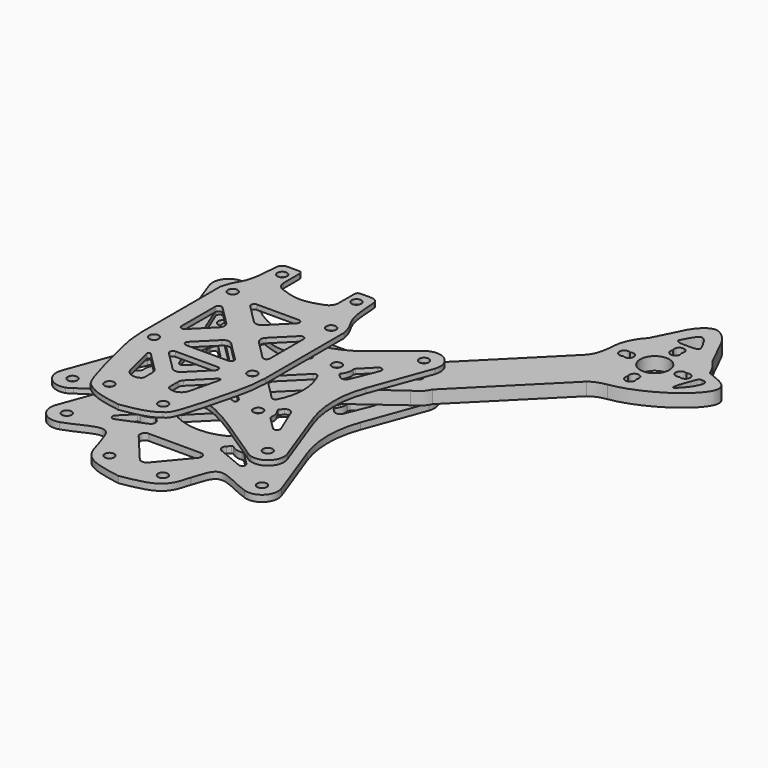
from build123d import *

# Parameters (mm, degrees)
F0_R     = 1.5
F2_DEPTH = 2
F4_START = 3
F1_R     = 1.5
F1_R_2   = 4.5
F4_DEPTH = 4
F7_START = 20
F6_R     = 1.5
F7_DEPTH = 1.5
F8_START = 9
F5_R     = 1.5
F8_DEPTH = 1.5


with BuildPart() as f2:
    # F0 (on Top) → F2 (new body)
    with BuildSketch(Plane.XY):
        with BuildLine():
            add(Edge.make_bspline(
                [(-28.6583371689, 34.989895508), (-15.5486081514, 28.1029236725), (-15.2531134537, 20.3288752095), (-15.0275822655, 35.7869570093)],
                knots=[0, 0, 0, 0, 13.3992828802, 13.3992828802, 13.3992828802, 13.3992828802], degree=3))
            ThreePointArc((-28.6583371689, 34.989895508), (-33.8221162144, 33.7485690999), (-34.9557615497, 28.560086322))
            Line((-34.9557615497, 28.560086322), (-28.2756954338, 10.3133747837))
            ThreePointArc((-28.2756954338, 10.3133747837), (-26.4471685044, -7.1088e-06), (-28.2756201348, -10.3134023513))
            Line((-28.2756201348, -10.3134023513), (-34.9643155344, -28.58409813))
            ThreePointArc((-34.9643155344, -28.58409813), (-33.8042341838, -33.7667341911), (-28.6341939914, -34.9817196608))
            add(Edge.make_bspline(
                [(-28.6341939914, -34.9817196608), (-24.495487875, -33.6930387827), (-16.3607874703, -27.7449542077), (-15.1366587225, -35.7631260416), (-14.33, -37.7577804035)],
                knots=[0, 0, 0, 0, 0.5615113554, 1, 1, 1, 1], degree=3))
            add(Edge.make_bspline(
                [(-14.33, -37.7577804035), (-13.6367446794, -40.3263257967), (-12.088150953, -46.0639424644), (-4.3010614265, -47.3817279873), (0, -48.1095835567)],
                knots=[0, 0, 0, 0, 0.447667654, 1, 1, 1, 1], degree=3))
            add(Edge.make_bspline(
                [(14.33, -37.7577804035), (13.6367446794, -40.3263257967), (12.088150953, -46.0639424644), (4.3010614265, -47.3817279873), (0, -48.1095835567)],
                knots=[0, 0, 0, 0, 0.447667654, 1, 1, 1, 1], degree=3))
            add(Edge.make_bspline(
                [(28.6583371689, -34.9898955092), (24.5097770544, -33.6967999), (16.3601661117, -27.7422129401), (15.1363049951, -35.7630085829), (14.33, -37.7577804035)],
                knots=[0, 0, 0, 0, 0.561784833, 1, 1, 1, 1], degree=3))
            ThreePointArc((28.6583371689, -34.9898955092), (33.8221162144, -33.748569101), (34.9557615497, -28.5600863232))
            Line((34.9557615497, -28.5600863232), (28.2756954338, -10.3133747849))
            ThreePointArc((28.2756954338, -10.3133747849), (26.4471685044, 7.1077e-06), (28.2756201348, 10.3134023502))
            Line((28.2756201348, 10.3134023502), (34.9643155344, 28.5840981288))
            ThreePointArc((34.9643155344, 28.5840981288), (33.8042341838, 33.76673419), (28.6341939914, 34.9817196596))
            add(Edge.make_bspline(
                [(15.0274820378, 35.7867377887), (15.2513136358, 20.3289797995), (15.5248044507, 28.1031931102), (28.6341939914, 34.9817196596)],
                knots=[0.5359060708, 0.5359060708, 0.5359060708, 0.5359060708, 13.9139411757, 13.9139411757, 13.9139411757, 13.9139411757], degree=3))
            ThreePointArc((15.0274820378, 35.7867377887), (14.4316299327, 37.1821951546), (13.0276916813, 37.7577804023))
            Line((13.0276916813, 37.7577804023), (-13.0277950954, 37.7577804023))
            ThreePointArc((-13.0277950954, 37.7577804023), (-14.4316552711, 37.1822721036), (-15.0275822655, 35.7869570093))
        make_face()
        with Locations((-30.25, -30.2500000006)):
            Circle(F0_R, mode=Mode.SUBTRACT)
        with Locations((-8.2733329443, -41.1618490551)):
            Circle(F0_R, mode=Mode.SUBTRACT)
        with BuildLine():
            ThreePointArc((-23.8517090122, -20.3161751069), (-25.1141961389, -20.4406647854), (-25.4828700073, -19.2268068843))
            Line((-25.4828700073, -19.2268068843), (-22.1833207357, -11.2506887671))
            ThreePointArc((-22.1833207357, -11.2506887671), (-21.0902108457, -10.3529698728), (-19.736579243, -10.7634207575))
            Line((-19.736579243, -10.7634207575), (-18.8553009264, -11.6446990741))
            ThreePointArc((-18.8553009264, -11.6446990741), (-18.7090370991, -11.9847340093), (-18.8367068235, -12.33217797))
            Line((-18.8367068235, -12.33217797), (-18.8542943682, -12.3517786311))
            ThreePointArc((-18.8542943682, -12.3517786311), (-19.6877326512, -13.9472514003), (-19.8489637612, -15.7400584892))
            Line((-19.8489637612, -15.7400584892), (-19.8303976916, -15.8549305034))
            ThreePointArc((-19.8303976916, -15.8549305034), (-19.8571321349, -16.2052315209), (-20.0404595752, -16.5049256699))
            Line((-20.0404595752, -16.5049256699), (-23.8517090122, -20.3161751069))
        make_face(mode=Mode.SUBTRACT)
        with BuildLine():
            Line((-11.2506887665, -22.1833207364), (-19.2268068836, -25.482870008))
            ThreePointArc((-19.2268068836, -25.482870008), (-20.4406647847, -25.1141961396), (-20.3161751062, -23.8517090128))
            Line((-20.3161751062, -23.8517090128), (-16.5049256693, -20.0404595759))
            ThreePointArc((-16.5049256693, -20.0404595759), (-16.2052315202, -19.8571321356), (-15.8549305027, -19.8303976923))
            Line((-15.8549305027, -19.8303976923), (-15.7400584885, -19.8489637619))
            ThreePointArc((-15.7400584885, -19.8489637619), (-13.9472513996, -19.6877326519), (-12.3517786304, -18.8542943689))
            Line((-12.3517786304, -18.8542943689), (-12.3321779693, -18.8367068242))
            ThreePointArc((-12.3321779693, -18.8367068242), (-11.9847340086, -18.7090370997), (-11.6446990734, -18.8553009271))
            Line((-11.6446990734, -18.8553009271), (-10.7634207569, -19.7365792436))
            ThreePointArc((-10.7634207569, -19.7365792436), (-10.3529698721, -21.0902108464), (-11.2506887665, -22.1833207364))
        make_face(mode=Mode.SUBTRACT)
        with Locations((-15.25, -15.2500000006)):
            Circle(F0_R, mode=Mode.SUBTRACT)
        with BuildLine():
            ThreePointArc((-7.7892382513, -15.2383616248), (-8.2896410828, -14.5053634666), (-8.0071487762, -13.6640030263))
            Line((-8.0071487762, -13.6640030263), (-1.4142135624, -7.0710678125))
            ThreePointArc((-1.4142135624, -7.0710678125), (0, -6.4852813748), (1.4142135624, -7.0710678125))
            Line((1.4142135624, -7.0710678125), (8.0039929944, -13.6608472445))
            ThreePointArc((8.0039929944, -13.6608472445), (8.287442711, -14.5050591849), (7.7853439372, -15.2405415869))
            Line((7.7853439372, -15.2405415869), (7.7684472975, -15.2500000006))
            ThreePointArc((7.7684472975, -15.2500000006), (0, -17.1146508417), (-7.7684472975, -15.2500000006))
            Line((-7.7684472975, -15.2500000006), (-7.7892382513, -15.2383616248))
        make_face(mode=Mode.SUBTRACT)
        with Locations((8.2733329443, -41.1618490551)):
            Circle(F0_R, mode=Mode.SUBTRACT)
        with BuildLine():
            Line((-1.3419338656, -38.0910861377), (-9.1892168108, -28.7161126104))
            ThreePointArc((-9.1892168108, -28.7161126104), (-9.3980668278, -27.118570832), (-8.0389877832, -26.2533181443))
            Line((-8.0389877832, -26.2533181443), (8.0389877833, -26.2533181443))
            ThreePointArc((8.0389877833, -26.2533181443), (9.398066828, -27.118570832), (9.189216811, -28.7161126104))
            Line((9.189216811, -28.7161126104), (1.3419338656, -38.0910861377))
            ThreePointArc((1.3419338656, -38.0910861377), (0, -38.7178259272), (-1.3419338656, -38.0910861377))
        make_face(mode=Mode.SUBTRACT)
        with Locations((30.25, -30.2500000006)):
            Circle(F0_R, mode=Mode.SUBTRACT)
        with BuildLine():
            ThreePointArc((20.3161751064, -23.8517090128), (20.4406647849, -25.1141961396), (19.2268068838, -25.482870008))
            Line((19.2268068838, -25.482870008), (11.2506887667, -22.1833207364))
            ThreePointArc((11.2506887667, -22.1833207364), (10.3529698723, -21.0902108464), (10.7634207571, -19.7365792436))
            Line((10.7634207571, -19.7365792436), (11.6446990736, -18.8553009271))
            ThreePointArc((11.6446990736, -18.8553009271), (11.9847340088, -18.7090370997), (12.3321779695, -18.8367068242))
            Line((12.3321779695, -18.8367068242), (12.3517786306, -18.8542943689))
            ThreePointArc((12.3517786306, -18.8542943689), (13.9472513998, -19.6877326519), (15.7400584887, -19.8489637619))
            Line((15.7400584887, -19.8489637619), (15.8549305029, -19.8303976923))
            ThreePointArc((15.8549305029, -19.8303976923), (16.2052315204, -19.8571321356), (16.5049256694, -20.0404595759))
            Line((16.5049256694, -20.0404595759), (20.3161751064, -23.8517090128))
        make_face(mode=Mode.SUBTRACT)
        with Locations((15.25, -15.2500000006)):
            Circle(F0_R, mode=Mode.SUBTRACT)
        with BuildLine():
            ThreePointArc((19.7365792431, -10.7634207575), (21.0902108459, -10.3529698728), (22.1833207359, -11.2506887671))
            Line((22.1833207359, -11.2506887671), (25.4828700075, -19.2268068842))
            ThreePointArc((25.4828700075, -19.2268068842), (25.1141961391, -20.4406647853), (23.8517090123, -20.3161751069))
            Line((23.8517090123, -20.3161751069), (20.0404595754, -16.5049256699))
            ThreePointArc((20.0404595754, -16.5049256699), (19.8571321351, -16.2052315209), (19.8303976918, -15.8549305033))
            Line((19.8303976918, -15.8549305033), (19.8489637614, -15.7400584892))
            ThreePointArc((19.8489637614, -15.7400584892), (19.6877326514, -13.9472514003), (18.8542943684, -12.3517786311))
            Line((18.8542943684, -12.3517786311), (18.8367068237, -12.33217797))
            ThreePointArc((18.8367068237, -12.33217797), (18.7090370992, -11.9847340093), (18.8553009266, -11.6446990741))
            Line((18.8553009266, -11.6446990741), (19.7365792431, -10.7634207575))
        make_face(mode=Mode.SUBTRACT)
        with BuildLine():
            ThreePointArc((-18.8367068237, 12.3321779688), (-18.7090370992, 11.9847340081), (-18.8553009266, 11.6446990729))
            Line((-18.8553009266, 11.6446990729), (-19.7365318181, 10.7634681813))
            ThreePointArc((-19.7365318181, 10.7634681813), (-21.0901735727, 10.3530193183), (-22.1832812244, 11.250755321))
            Line((-22.1832812244, 11.250755321), (-25.4825410679, 19.2264854211))
            ThreePointArc((-25.4825410679, 19.2264854211), (-25.1138561851, 20.4403344014), (-23.851374797, 20.3158408904))
            Line((-23.851374797, 20.3158408904), (-20.0404595754, 16.5049256687))
            ThreePointArc((-20.0404595754, 16.5049256687), (-19.8571321351, 16.2052315197), (-19.8303976918, 15.8549305022))
            Line((-19.8303976918, 15.8549305022), (-19.8489637614, 15.740058488))
            ThreePointArc((-19.8489637614, 15.740058488), (-19.6877326514, 13.9472513991), (-18.8542943684, 12.3517786299))
            Line((-18.8542943684, 12.3517786299), (-18.8367068237, 12.3321779688))
        make_face(mode=Mode.SUBTRACT)
        with BuildLine():
            ThreePointArc((-13.6608472446, -8.003992994), (-14.505059185, -8.2874427105), (-15.2405415869, -7.7853439367))
            Line((-15.2405415869, -7.7853439367), (-15.25, -7.7684472983))
            ThreePointArc((-15.25, -7.7684472983), (-17.1146508411, -6e-10), (-15.25, 7.7684472971))
            Line((-15.25, 7.7684472971), (-15.2405415859, 7.7853439372))
            ThreePointArc((-15.2405415859, 7.7853439372), (-14.505059184, 8.2874427111), (-13.6608472436, 8.0039929945))
            Line((-13.6608472436, 8.0039929945), (-7.0710678122, 1.4142135631))
            ThreePointArc((-7.0710678122, 1.4142135631), (-6.4852813746, 7e-10), (-7.0710678122, -1.4142135616))
            Line((-7.0710678122, -1.4142135616), (-13.6608472446, -8.003992994))
        make_face(mode=Mode.SUBTRACT)
        with Locations((-15.25, 15.2499999994)):
            Circle(F0_R, mode=Mode.SUBTRACT)
        with BuildLine():
            ThreePointArc((7.7853439372, 15.2405415857), (8.287442711, 14.5050591838), (8.0039929944, 13.6608472433))
            Line((8.0039929944, 13.6608472433), (1.4142135624, 7.0710678113))
            ThreePointArc((1.4142135624, 7.0710678113), (0, 6.4852813737), (-1.4142135624, 7.0710678113))
            Line((-1.4142135624, 7.0710678113), (-8.0039929944, 13.6608472433))
            ThreePointArc((-8.0039929944, 13.6608472433), (-8.287442711, 14.5050591838), (-7.7853439372, 15.2405415857))
            Line((-7.7853439372, 15.2405415857), (-7.7684472975, 15.2499999994))
            ThreePointArc((-7.7684472975, 15.2499999994), (0, 17.1146508406), (7.7684472975, 15.2499999994))
            Line((7.7684472975, 15.2499999994), (7.7853439372, 15.2405415857))
        make_face(mode=Mode.SUBTRACT)
        with Locations((-30.25, 30.2499999994)):
            Circle(F0_R, mode=Mode.SUBTRACT)
        with BuildLine():
            ThreePointArc((-7.7684472975, 20.1190513336), (-9.4080907996, 20.7386520685), (-8.9382902045, 22.4273270773))
            Line((-8.9382902045, 22.4273270773), (-1.06072927, 27.355528746))
            ThreePointArc((-1.06072927, 27.355528746), (0, 27.6599894761), (1.0607292699, 27.355528746))
            Line((1.0607292699, 27.355528746), (8.9382902045, 22.4273270773))
            ThreePointArc((8.9382902045, 22.4273270773), (9.4121452662, 20.7467816187), (7.7853439372, 20.1125189809))
            ThreePointArc((7.7853439372, 20.1125189809), (0.0090577048, 21.5667549236), (-7.7684472975, 20.1190513336))
        make_face(mode=Mode.SUBTRACT)
        with Locations((-11.5, 29.7577804023)):
            Circle(F0_R, mode=Mode.SUBTRACT)
        with BuildLine():
            Line((7.0710678124, 1.4142135624), (13.6608472439, 8.0039929938))
            ThreePointArc((13.6608472439, 8.0039929938), (14.5050591843, 8.2874427104), (15.2405415863, 7.7853439366))
            Line((15.2405415863, 7.7853439366), (15.25, 7.7684472971))
            ThreePointArc((15.25, 7.7684472971), (17.1146508411, -6e-10), (15.25, -7.7684472983))
            Line((15.25, -7.7684472983), (15.2405415867, -7.7853439371))
            ThreePointArc((15.2405415867, -7.7853439371), (14.5050591848, -8.2874427109), (13.6608472444, -8.0039929943))
            Line((13.6608472444, -8.0039929943), (7.0710678124, -1.4142135624))
            ThreePointArc((7.0710678124, -1.4142135624), (6.4852813748, 0), (7.0710678124, 1.4142135624))
        make_face(mode=Mode.SUBTRACT)
        with Locations((15.25, 15.2499999994)):
            Circle(F0_R, mode=Mode.SUBTRACT)
        with BuildLine():
            Line((19.8247048971, 15.785759925), (19.8053184489, 15.9004963368))
            ThreePointArc((19.8053184489, 15.9004963368), (19.8295490283, 16.2509794496), (20.0107302331, 16.5519759685))
            Line((20.0107302331, 16.5519759685), (23.8084562188, 20.4043695836))
            ThreePointArc((23.8084562188, 20.4043695836), (25.0693920791, 20.5382911332), (25.4479247727, 19.3280815542))
            Line((25.4479247727, 19.3280815542), (22.2099579078, 11.3050038785))
            ThreePointArc((22.2099579078, 11.3050038785), (21.1235499455, 10.3976310998), (19.7659136105, 10.7981697397))
            Line((19.7659136105, 10.7981697397), (18.8636878016, 11.6875924575))
            ThreePointArc((18.8636878016, 11.6875924575), (18.7150078324, 12.0262851571), (18.8397994936, 12.37448843))
            Line((18.8397994936, 12.37448843), (18.8575858105, 12.3946446988))
            ThreePointArc((18.8575858105, 12.3946446988), (19.6770217108, 13.9944130467), (19.8247048971, 15.785759925))
        make_face(mode=Mode.SUBTRACT)
        with Locations((11.5, 29.7577804023)):
            Circle(F0_R, mode=Mode.SUBTRACT)
        with Locations((30.25, 30.2499999994)):
            Circle(F0_R, mode=Mode.SUBTRACT)
    extrude(amount=F2_DEPTH)


with BuildPart() as f4:
    # F1 (on Top) → F4 (new body)
    with BuildSketch(Plane.XY.offset(F4_START)):
        with BuildLine():
            add(Edge.make_bspline(
                [(53.8403756487, 63.7304752458), (55.416769934, 65.2037108877), (56.4797969246, 66.7322054505), (56.9693953395, 70.96)],
                knots=[0, 0, 0, 0, 7.8776133694, 7.8776133694, 7.8776133694, 7.8776133694], degree=3))
            Line((53.8403756487, 63.7304752458), (27.2135911477, 37.1036907448))
            ThreePointArc((27.2135911477, 37.1036907448), (24.9560944806, 35.5533008589), (23.4057045947, 33.2958041918))
            Line((23.4057045947, 33.2958041918), (13.6185183249, 19.9730840161))
            ThreePointArc((13.6185183249, 19.9730840161), (11.3998018999, 18.428606374), (10.3093393921, 15.9549440526))
            Line((10.3093393921, 15.9549440526), (6.3693953395, 12.015))
            Line((6.3693953395, 12.015), (0.0093953395, 5.655))
            Line((0.0093953395, 5.655), (0.0093953395, 0))
            Line((0.0093953395, 0), (5.6643953395, 0))
            Line((5.6643953395, 0), (12.0243953395, 6.36))
            Line((12.0243953395, 6.36), (15.964339392, 10.2999440526))
            ThreePointArc((15.964339392, 10.2999440526), (18.4380017135, 11.3904065604), (19.9824793556, 13.6091229854))
            Line((19.9824793556, 13.6091229854), (33.3051995313, 23.3963092552))
            ThreePointArc((33.3051995313, 23.3963092552), (35.5626961984, 24.9466991411), (37.1130860843, 27.2041958082))
            Line((37.1130860843, 27.2041958082), (63.6551645076, 53.7462742315))
            add(Edge.make_bspline(
                [(63.6551645076, 53.7462742315), (65.3627067804, 54.9906902015), (66.7258799076, 55.3231723607), (68.4891356677, 55.6597283697)],
                knots=[0, 0, 0, 0, 5.1989021836, 5.1989021836, 5.1989021836, 5.1989021836], degree=3))
            add(Edge.make_bspline(
                [(84.0894447875, 75.8451102834), (87.0090253606, 74.6406662064), (97.809192454, 71.4575524374), (79.1750401258, 57.3118105531), (68.4891356677, 55.6597283697)],
                knots=[0, 0, 0, 0, 0.3577567319, 1, 1, 1, 1], degree=3))
            ThreePointArc((84.0894447875, 75.8451102834), (82.7490756952, 78.5256546787), (80.8688902761, 80.8594949366))
            Line((80.8688902761, 80.8594949366), (76.2193953395, 90.2586398484))
            add(Edge.make_bspline(
                [(65.7193953395, 90.2586398484), (67.2193953395, 92.6020138718), (70.9693953395, 96.3179861282), (74.7193953395, 92.6020138718), (76.2193953395, 90.2586398484)],
                knots=[0, 0, 0, 0, 0.5, 1, 1, 1, 1], degree=3))
            Line((65.7193953395, 90.2586398484), (61.0699004029, 80.8594949366))
            ThreePointArc((61.0699004029, 80.8594949366), (58.0350818843, 76.3175680531), (56.9693953395, 70.96))
        make_face()
        with Locations((15.2593953395, 15.25)):
            Circle(F1_R, mode=Mode.SUBTRACT)
        with Locations((30.2593953395, 30.25)):
            Circle(F1_R, mode=Mode.SUBTRACT)
        with BuildLine():
            ThreePointArc((72.2684334452, 62.21), (70.9693953395, 59.96), (69.6703572338, 62.21))
            ThreePointArc((69.6703572338, 62.21), (70.9693953395, 64.46), (72.2684334452, 62.21))
        make_face(mode=Mode.SUBTRACT)
        with BuildLine():
            ThreePointArc((62.2193953395, 72.2590381057), (64.4693953395, 70.96), (62.2193953395, 69.6609618943))
            ThreePointArc((62.2193953395, 69.6609618943), (59.9693953395, 70.96), (62.2193953395, 72.2590381057))
        make_face(mode=Mode.SUBTRACT)
        with Locations((70.9693953395, 70.96)):
            Circle(F1_R_2, mode=Mode.SUBTRACT)
        with BuildLine():
            add(Edge.make_bspline(
                [(82.4060514569, 64.5534098148), (80.7914603636, 63.0556593791), (83.9801204568, 71.8950702465), (84.2074600213, 71.8239934193), (84.9451732404, 71.783184101)],
                knots=[0, 0, 0, 0, 0.6805312174, 1, 1, 1, 1], degree=3))
            add(Edge.make_bspline(
                [(84.9451732404, 71.783184101), (85.7962933376, 71.6849426877), (87.6041236849, 71.2964912458), (84.6678863419, 66.376809069), (82.4060514569, 64.5534098148)],
                knots=[0, 0, 0, 0, 0.32334118, 1, 1, 1, 1], degree=3))
        make_face(mode=Mode.SUBTRACT)
        with BuildLine():
            ThreePointArc((79.7193953395, 69.6609618943), (77.4693953395, 70.96), (79.7193953395, 72.2590381057))
            ThreePointArc((79.7193953395, 72.2590381057), (81.9693953395, 70.96), (79.7193953395, 69.6609618943))
        make_face(mode=Mode.SUBTRACT)
        with BuildLine():
            ThreePointArc((72.2684334452, 79.71), (70.9693953395, 77.46), (69.6703572338, 79.71))
            ThreePointArc((69.6703572338, 79.71), (70.9693953395, 81.96), (72.2684334452, 79.71))
        make_face(mode=Mode.SUBTRACT)
        with BuildLine():
            add(Edge.make_bspline(
                [(67.4763052703, 84.5172239698), (67.595660109, 83.524372308), (70.9693953395, 83.524372308), (74.34313057, 83.524372308), (74.4624854087, 84.5172239698)],
                knots=[0, 0, 0, 0, 0.5, 1, 1, 1, 1], degree=3))
            add(Edge.make_bspline(
                [(67.4763052703, 84.5172239698), (68.6406686267, 86.8665499989), (70.9693953395, 91.5652020569), (73.2981220523, 86.8665499989), (74.4624854087, 84.5172239698)],
                knots=[0, 0, 0, 0, 0.5, 1, 1, 1, 1], degree=3))
        make_face(mode=Mode.SUBTRACT)
    extrude(amount=F4_DEPTH)


with BuildPart() as f7:
    # F6 (on Top) → F7 (new body)
    with BuildSketch(Plane.XY.offset(F7_START)):
        with BuildLine():
            add(Edge.make_bspline(
                [(-19.25, -15.2218541075), (-19.0684905374, -19.7268529833), (-17.9623264747, -24.6907042809), (-13.2785718821, -43.084666195), (-11.6053951728, -44.1968771124), (-11.0003547743, -44.5749795424)],
                knots=[0, 0, 0, 0, 0.3683029461, 0.8298524693, 1, 1, 1, 1], degree=3))
            add(Edge.make_bspline(
                [(-11.0003547743, -44.5749795424), (-7.8986920416, -46.9837644324), (-3.9995196275, -47.3454079802), (0, -48.1093942399)],
                knots=[0, 0, 0, 0, 11.5542153526, 11.5542153526, 11.5542153526, 11.5542153526], degree=3))
            add(Edge.make_bspline(
                [(11.0003547743, -44.5749795424), (7.8986920416, -46.9837644324), (3.9995196275, -47.3454079802), (0, -48.1093942399)],
                knots=[0, 0, 0, 0, 11.5542153526, 11.5542153526, 11.5542153526, 11.5542153526], degree=3))
            add(Edge.make_bspline(
                [(19.25, -15.2218541075), (19.0667337669, -19.7267716154), (17.9562925595, -24.6902276301), (13.2790290127, -43.0847539077), (11.6055152346, -44.1969091306), (11.0003547743, -44.5749795424)],
                knots=[0, 0, 0, 0, 0.368314136, 0.829851714, 1, 1, 1, 1], degree=3))
            Line((19.25, -15.2218541075), (19.25, 15.2781458925))
            add(Edge.make_bspline(
                [(15.0790967662, 31.8597836794), (15.7273210805, 18.4148469189), (17.670676786, 22.4575338068), (19.25, 15.2781458925)],
                knots=[0.8128411452, 0.8128411452, 0.8128411452, 0.8128411452, 18.97635654, 18.97635654, 18.97635654, 18.97635654], degree=3))
            ThreePointArc((15.0790967662, 31.8597836794), (14.4611582834, 33.211334576), (13.0814172406, 33.7634690247))
            add(Edge.make_bspline(
                [(9.5020394819, 33.7713114856), (10.6902314797, 33.7688881845), (11.9558724743, 33.7634690247), (13.0814172406, 33.7634690247)],
                knots=[1.0243447025, 1.0243447025, 1.0243447025, 1.0243447025, 4.5814260604, 4.5814260604, 4.5814260604, 4.5814260604], degree=3))
            ThreePointArc((9.5020394819, 33.7713114856), (8.7936146526, 33.479141045), (8.5, 32.7713135654))
            add(Edge.make_bspline(
                [(8.5, 32.285449478), (8.5, 32.4472244474), (8.5, 32.609243629), (8.5, 32.7713135654)],
                knots=[0.2605482636, 0.2605482636, 0.2605482636, 0.2605482636, 0.7461719983, 0.7461719983, 0.7461719983, 0.7461719983], degree=3))
            add(Edge.make_bspline(
                [(8.5, 32.025302314), (8.5, 32.1119278185), (8.5, 32.1986534992), (8.5, 32.285449478)],
                knots=[0, 0, 0, 0, 0.2605482636, 0.2605482636, 0.2605482636, 0.2605482636], degree=3))
            Line((8.5, 32.025302314), (8.5, 26.5908181775))
            ThreePointArc((8.5, 26.5908181775), (7.9671627129, 24.8840351954), (6.5579279014, 23.7835439559))
            add(Edge.make_bspline(
                [(-6.5579279014, 23.7835439559), (-4.3358517051, 22.9461493085), (0, 21.578151535), (4.3358517051, 22.9461493085), (6.5579279014, 23.7835439559)],
                knots=[0.1121315865, 0.1121315865, 0.1121315865, 0.1121315865, 0.5, 0.8878684135, 0.8878684135, 0.8878684135, 0.8878684135], degree=3))
            ThreePointArc((-6.5579279014, 23.7835439559), (-7.9671627129, 24.8840351954), (-8.5, 26.5908181775))
            Line((-8.5, 26.5908181775), (-8.5, 32.025302314))
            add(Edge.make_bspline(
                [(-8.5, 32.025302314), (-8.5, 32.1119278185), (-8.5, 32.1986534992), (-8.5, 32.285449478)],
                knots=[0, 0, 0, 0, 0.2605482636, 0.2605482636, 0.2605482636, 0.2605482636], degree=3))
            add(Edge.make_bspline(
                [(-8.5, 32.285449478), (-8.5, 32.4469519552), (-8.5, 32.6086978226), (-8.5, 32.7704945986)],
                knots=[0.2605482636, 0.2605482636, 0.2605482636, 0.2605482636, 0.7453540183, 0.7453540183, 0.7453540183, 0.7453540183], degree=3))
            ThreePointArc((-8.5, 32.7704945986), (-8.7935873047, 33.4782947851), (-9.501962208, 33.7704926735))
            Line((-9.501962208, 33.7704926735), (-13.0814172406, 33.7634690247))
            ThreePointArc((-13.0814172406, 33.7634690247), (-14.4611582834, 33.211334576), (-15.0790967662, 31.8597836794))
            add(Edge.make_bspline(
                [(-15.0790967662, 31.8597836794), (-15.7273210805, 18.4148469189), (-17.670676786, 22.4575338068), (-19.25, 15.2781458925)],
                knots=[0.8128411452, 0.8128411452, 0.8128411452, 0.8128411452, 18.97635654, 18.97635654, 18.97635654, 18.97635654], degree=3))
            Line((-19.25, 15.2781458925), (-19.25, -15.2218541075))
        make_face()
        with Locations((-8.3293477558, -41.1257331912)):
            Circle(F6_R, mode=Mode.SUBTRACT)
        with BuildLine():
            ThreePointArc((-11.2741795299, -22.9536277928), (-11.0338873267, -22.3989447209), (-10.4349964383, -22.4810626653))
            Line((-10.4349964383, -22.4810626653), (-4.5076118446, -28.408447259))
            ThreePointArc((-4.5076118446, -28.408447259), (-4.0740663419, -29.0572939567), (-3.9218254069, -29.8226608214))
            Line((-3.9218254069, -29.8226608214), (-3.9218254069, -32.9968597055))
            ThreePointArc((-3.9218254069, -32.9968597055), (-4.0264596985, -33.4421913215), (-4.3184659033, -33.7943290211))
            Line((-4.3184659033, -33.7943290211), (-4.4003069963, -33.8562493989))
            ThreePointArc((-4.4003069963, -33.8562493989), (-7.223873087, -34.0855754205), (-9.0722171951, -31.9387778169))
            Line((-9.0722171951, -31.9387778169), (-11.2741795299, -22.9536277928))
        make_face(mode=Mode.SUBTRACT)
        with Locations((-15.25, -15.2218541075)):
            Circle(F6_R, mode=Mode.SUBTRACT)
        with Locations((8.3288047093, -41.1259644251)):
            Circle(F6_R, mode=Mode.SUBTRACT)
        with BuildLine():
            Line((4.5076118446, -28.408447259), (10.4349123369, -22.4811467667))
            ThreePointArc((10.4349123369, -22.4811467667), (11.0338107336, -22.3990330505), (11.2740913261, -22.9537286326))
            Line((11.2740913261, -22.9537286326), (9.0718254069, -31.9387778169))
            ThreePointArc((9.0718254069, -31.9387778169), (7.2237469097, -34.0856955052), (4.4002690575, -33.8562995378))
            Line((4.4002690575, -33.8562995378), (4.3183823385, -33.7943311455))
            ThreePointArc((4.3183823385, -33.7943311455), (4.0264363662, -33.4422097633), (3.9218254069, -32.9969250614))
            Line((3.9218254069, -32.9969250614), (3.9218254069, -29.8226608214))
            ThreePointArc((3.9218254069, -29.8226608214), (4.0740663419, -29.0572939567), (4.5076118446, -28.408447259))
        make_face(mode=Mode.SUBTRACT)
        with BuildLine():
            Line((-1.4142135624, -25.3091152098), (-7.2178932188, -19.5054355534))
            ThreePointArc((-7.2178932188, -19.5054355534), (-7.4346659701, -18.4156453398), (-6.5107864376, -17.7983287722))
            Line((-6.5107864376, -17.7983287722), (6.5107864376, -17.7983287722))
            ThreePointArc((6.5107864376, -17.7983287722), (7.4346659701, -18.4156453398), (7.2178932188, -19.5054355534))
            Line((7.2178932188, -19.5054355534), (1.4142135624, -25.3091152098))
            ThreePointArc((1.4142135624, -25.3091152098), (0, -25.8949016474), (-1.4142135624, -25.3091152098))
        make_face(mode=Mode.SUBTRACT)
        with BuildLine():
            ThreePointArc((-1.4142135624, -6.1360676699), (0, -5.5502812323), (1.4142135624, -6.1360676699))
            Line((1.4142135624, -6.1360676699), (7.2178932188, -11.9397473263))
            ThreePointArc((7.2178932188, -11.9397473263), (7.4346659701, -13.0295375399), (6.5107864376, -13.6468541075))
            Line((6.5107864376, -13.6468541075), (-6.5107864376, -13.6468541075))
            ThreePointArc((-6.5107864376, -13.6468541075), (-7.4346659701, -13.0295375399), (-7.2178932188, -11.9397473263))
            Line((-7.2178932188, -11.9397473263), (-1.4142135624, -6.1360676699))
        make_face(mode=Mode.SUBTRACT)
        with Locations((15.25, -15.2218541075)):
            Circle(F6_R, mode=Mode.SUBTRACT)
        with BuildLine():
            Line((-11.9678932188, 7.2460391113), (-6.1642135624, 1.4423594549))
            ThreePointArc((-6.1642135624, 1.4423594549), (-5.5784271247, 0.0281458925), (-6.1642135624, -1.3860676699))
            Line((-6.1642135624, -1.3860676699), (-11.9678932188, -7.1897473263))
            ThreePointArc((-11.9678932188, -7.1897473263), (-13.0576834324, -7.4065200777), (-13.675, -6.4826405451))
            Line((-13.675, -6.4826405451), (-13.675, 6.5389323301))
            ThreePointArc((-13.675, 6.5389323301), (-13.0576834324, 7.4628118626), (-11.9678932188, 7.2460391113))
        make_face(mode=Mode.SUBTRACT)
        with Locations((-15.25, 15.2781458925)):
            Circle(F6_R, mode=Mode.SUBTRACT)
        with Locations((-11.499689569, 29.7634854823)):
            Circle(F6_R, mode=Mode.SUBTRACT)
        with BuildLine():
            ThreePointArc((1.4142135624, 6.1923594549), (0, 5.6065730172), (-1.4142135624, 6.1923594549))
            Line((-1.4142135624, 6.1923594549), (-7.2178932188, 11.9960391113))
            ThreePointArc((-7.2178932188, 11.9960391113), (-7.4346659701, 13.0858293249), (-6.5107864376, 13.7031458925))
            Line((-6.5107864376, 13.7031458925), (6.5107864376, 13.7031458925))
            ThreePointArc((6.5107864376, 13.7031458925), (7.4346659701, 13.0858293249), (7.2178932188, 11.9960391113))
            Line((7.2178932188, 11.9960391113), (1.4142135624, 6.1923594549))
        make_face(mode=Mode.SUBTRACT)
        with BuildLine():
            Line((11.9678932188, -7.1897473263), (6.1642135624, -1.3860676699))
            ThreePointArc((6.1642135624, -1.3860676699), (5.5784271247, 0.0281458925), (6.1642135624, 1.4423594549))
            Line((6.1642135624, 1.4423594549), (11.9678932188, 7.2460391113))
            ThreePointArc((11.9678932188, 7.2460391113), (13.0576834324, 7.4628118626), (13.675, 6.5389323301))
            Line((13.675, 6.5389323301), (13.675, -6.4826405451))
            ThreePointArc((13.675, -6.4826405451), (13.0576834324, -7.4065200777), (11.9678932188, -7.1897473263))
        make_face(mode=Mode.SUBTRACT)
        with Locations((15.25, 15.2781458925)):
            Circle(F6_R, mode=Mode.SUBTRACT)
        with Locations((11.499689569, 29.7634854822)):
            Circle(F6_R, mode=Mode.SUBTRACT)
    extrude(amount=F7_DEPTH)


with BuildPart() as f8:
    # F5 (on Top) → F8 (new body)
    with BuildSketch(Plane.XY.offset(F8_START)):
        with BuildLine():
            ThreePointArc((-26.9407032856, 36.2600348998), (-27.7551557637, 36.8489935616), (-28.6709446924, 37.2631623465))
            ThreePointArc((-28.6709446924, 37.2631623465), (-33.8348197995, 36.0222356117), (-34.9688667131, 30.8338405921))
            Line((-34.9688667131, 30.8338405921), (-28.2886697962, 12.5867673035))
            ThreePointArc((-28.2886697962, 12.5867673035), (-26.4601436815, 2.2733832229), (-28.2885975317, -8.0400136697))
            Line((-28.2885975317, -8.0400136697), (-34.9770950156, -26.3101566446))
            ThreePointArc((-34.9770950156, -26.3101566446), (-33.8176199057, -31.4929283694), (-28.6477218702, -32.7085185901))
            ThreePointArc((-28.6477218702, -32.7085185901), (-27.7339748711, -32.2898641192), (-26.9224202046, -31.6969187864))
            Line((-26.9224202046, -31.6969187864), (-15.2629743804, -23.98008234))
            add(Edge.make_bspline(
                [(-15.2629743804, -23.98008234), (-10.179641047, -20.7141435083), (-0.0129743803, -14.1822658449), (10.1536922863, -20.7141435083), (15.2370256196, -23.98008234)],
                knots=[0, 0, 0, 0, 0.5, 1, 1, 1, 1], degree=3))
            Line((15.2370256196, -23.98008234), (26.9147545249, -31.7132548104))
            ThreePointArc((26.9147545249, -31.7132548104), (27.7292070029, -32.3022134723), (28.6449959317, -32.7163822571))
            ThreePointArc((28.6449959317, -32.7163822571), (33.8088710387, -31.4754555224), (34.9429179524, -26.2870605027))
            Line((34.9429179524, -26.2870605027), (28.2627210354, -8.0399872141))
            ThreePointArc((28.2627210354, -8.0399872141), (26.4341949208, 2.2733968665), (28.2626487709, 12.586793759))
            Line((28.2626487709, 12.586793759), (34.9511462548, 30.8569367339))
            ThreePointArc((34.9511462548, 30.8569367339), (33.7916711449, 36.0397084588), (28.6217731094, 37.2552986795))
            ThreePointArc((28.6217731094, 37.2552986795), (27.7080261104, 36.8366442085), (26.8964714439, 36.2436988758))
            Line((26.8964714439, 36.2436988758), (15.2212491446, 26.7733900447))
            add(Edge.make_bspline(
                [(-15.2787508554, 26.7733900447), (-10.8797858751, 23.8265282552), (-0.0532688862, 20.1720392091), (10.8797858751, 23.8112762216), (15.2212491446, 26.7733900447)],
                knots=[0, 0, 0, 0, 0.5000467941, 1, 1, 1, 1], degree=3))
            Line((-15.2787508554, 26.7733900447), (-26.9407032856, 36.2600348998))
        make_face()
        with Locations((-30.2629743804, -27.9766099553)):
            Circle(F5_R, mode=Mode.SUBTRACT)
        with BuildLine():
            ThreePointArc((-23.8489069176, -18.0427905908), (-25.1113940444, -18.1672802692), (-25.4800679128, -16.9534223681))
            Line((-25.4800679128, -16.9534223681), (-22.1805186412, -8.977304251))
            ThreePointArc((-22.1805186412, -8.977304251), (-21.0874087512, -8.0795853567), (-19.7337771484, -8.4900362414))
            Line((-19.7337771484, -8.4900362414), (-18.8524988319, -9.3713145579))
            ThreePointArc((-18.8524988319, -9.3713145579), (-18.7062350045, -9.7113494932), (-18.833904729, -10.0587934538))
            Line((-18.833904729, -10.0587934538), (-18.8514922737, -10.0783941149))
            ThreePointArc((-18.8514922737, -10.0783941149), (-19.6849305567, -11.6738668841), (-19.8461616667, -13.466673973))
            Line((-19.8461616667, -13.466673973), (-19.8275955971, -13.5815459872))
            ThreePointArc((-19.8275955971, -13.5815459872), (-19.8543300404, -13.9318470047), (-20.0376574807, -14.2315411538))
            Line((-20.0376574807, -14.2315411538), (-23.8489069176, -18.0427905908))
        make_face(mode=Mode.SUBTRACT)
        with Locations((-15.2471979054, -12.9766154845)):
            Circle(F5_R, mode=Mode.SUBTRACT)
        with BuildLine():
            ThreePointArc((-13.6600131315, -5.726668306), (-14.5041657047, -6.0102947774), (-15.2397532199, -5.5083500098))
            Line((-15.2397532199, -5.5083500098), (-15.2471979054, -5.4950572526))
            ThreePointArc((-15.2471979054, -5.4950572526), (-17.1135691016, 2.2733900447), (-15.2471979054, 10.041837342))
            Line((-15.2471979054, 10.041837342), (-15.24273859, 10.0498062874))
            ThreePointArc((-15.24273859, 10.0498062874), (-14.5073304159, 10.552013774), (-13.6630765854, 10.2686888511))
            Line((-13.6630765854, 10.2686888511), (-7.0780798423, 3.683692108))
            ThreePointArc((-7.0780798423, 3.683692108), (-6.4922934046, 2.2694785456), (-7.0780798423, 0.8552649832))
            Line((-7.0780798423, 0.8552649832), (-13.6600131315, -5.726668306))
        make_face(mode=Mode.SUBTRACT)
        with Locations((30.2370256196, -27.9766099553)):
            Circle(F5_R, mode=Mode.SUBTRACT)
        with BuildLine():
            ThreePointArc((-7.7816537569, -12.9591669623), (-8.2829493322, -12.2265343934), (-8.001034186, -11.3847674512))
            Line((-8.001034186, -11.3847674512), (-1.427727924, -4.8034136383))
            ThreePointArc((-1.427727924, -4.8034136383), (-0.0138729894, -4.2167621451), (1.4006986714, -4.801683308))
            Line((1.4006986714, -4.801683308), (7.9815684526, -11.37450613))
            ThreePointArc((7.9815684526, -11.37450613), (8.2654849902, -12.2193895506), (7.7626098224, -12.9552925065))
            Line((7.7626098224, -12.9552925065), (7.7244458087, -12.9766154845))
            add(Edge.make_bspline(
                [(-7.7503945694, -12.9766154845), (-5.1645959639, -11.9759777802), (0.0020637685, -9.9766130491), (5.1519589479, -11.9772519711), (7.7244458087, -12.9766154845)],
                knots=[0, 0, 0, 0, 0.5004778212, 1, 1, 1, 1], degree=3))
            Line((-7.7503945694, -12.9766154845), (-7.7816537569, -12.9591669623))
        make_face(mode=Mode.SUBTRACT)
        with Locations((15.2528020946, -12.9766154845)):
            Circle(F5_R, mode=Mode.SUBTRACT)
        with BuildLine():
            Line((7.0557704686, 3.6852806441), (13.6380885864, 10.267598762))
            ThreePointArc((13.6380885864, 10.267598762), (14.4819467408, 10.5509556529), (15.2171693716, 10.0491236138))
            Line((15.2171693716, 10.0491236138), (15.2212491446, 10.041837342))
            ThreePointArc((15.2212491446, 10.041837342), (17.0876203409, 2.2733900447), (15.2212491446, -5.4950572526))
            Line((15.2212491446, -5.4950572526), (15.2156406206, -5.5050714767))
            ThreePointArc((15.2156406206, -5.5050714767), (14.4802031371, -6.0069702904), (13.6361480691, -5.7235240811))
            Line((13.6361480691, -5.7235240811), (7.0557704686, 0.8568535194))
            ThreePointArc((7.0557704686, 0.8568535194), (6.4699840309, 2.2710670817), (7.0557704686, 3.6852806441))
        make_face(mode=Mode.SUBTRACT)
        with BuildLine():
            ThreePointArc((19.7370620173, -8.4877181194), (21.0904813131, -8.0765677155), (22.1840550096, -8.9737215569))
            Line((22.1840550096, -8.9737215569), (25.4877259998, -16.9481333598))
            ThreePointArc((25.4877259998, -16.9481333598), (25.1196795178, -18.1621816342), (23.8571282218, -18.0383444417))
            Line((23.8571282218, -18.0383444417), (20.0439095917, -14.2290652158))
            ThreePointArc((20.0439095917, -14.2290652158), (19.8604272901, -13.9294658528), (19.8335118104, -13.5791786987))
            Line((19.8335118104, -13.5791786987), (19.8520185102, -13.4642971047))
            ThreePointArc((19.8520185102, -13.4642971047), (19.6898608763, -11.6715735815), (18.855598144, -10.0765317569))
            Line((18.855598144, -10.0765317569), (18.8380004718, -10.0569401879))
            ThreePointArc((18.8380004718, -10.0569401879), (18.7101512009, -9.7095622549), (18.8562392743, -9.3694517741))
            Line((18.8562392743, -9.3694517741), (19.7370620173, -8.4877181194))
        make_face(mode=Mode.SUBTRACT)
        with BuildLine():
            ThreePointArc((-18.8639492325, 14.6037202772), (-18.7360999616, 14.2563423443), (-18.8821880351, 13.9162318635))
            Line((-18.8821880351, 13.9162318635), (-19.7625740111, 13.0349354275))
            ThreePointArc((-19.7625740111, 13.0349354275), (-21.1161701038, 12.6238201487), (-22.2097049426, 13.5212719362))
            Line((-22.2097049426, 13.5212719362), (-25.5088845668, 21.4902583872))
            ThreePointArc((-25.5088845668, 21.4902583872), (-25.1406462244, 22.7041513988), (-23.8781948293, 22.5802474216))
            Line((-23.8781948293, 22.5802474216), (-20.0698583524, 18.7758453052))
            ThreePointArc((-20.0698583524, 18.7758453052), (-19.8863760509, 18.4762459421), (-19.8594605711, 18.1259587881))
            Line((-19.8594605711, 18.1259587881), (-19.8779672709, 18.0110771941))
            ThreePointArc((-19.8779672709, 18.0110771941), (-19.715809637, 16.2183536709), (-18.8815469047, 14.6233118463))
            Line((-18.8815469047, 14.6233118463), (-18.8639492325, 14.6037202772))
        make_face(mode=Mode.SUBTRACT)
        with Locations((-15.2787508554, 17.5233955738)):
            Circle(F5_R, mode=Mode.SUBTRACT)
        with BuildLine():
            ThreePointArc((7.7605848203, 17.5032086885), (8.263364843, 16.7678034482), (7.9800046348, 15.9232233093))
            Line((7.9800046348, 15.9232233093), (1.3989162185, 9.342134893))
            ThreePointArc((1.3989162185, 9.342134893), (-0.0152973439, 8.7563484554), (-1.4295109063, 9.342134893))
            Line((-1.4295109063, 9.342134893), (-8.0086569305, 15.9212809173))
            ThreePointArc((-8.0086569305, 15.9212809173), (-8.2921069909, 16.7660596794), (-7.7892590642, 17.5016812234))
            Line((-7.7892590642, 17.5016812234), (-7.7503945694, 17.5233955738))
            add(Edge.make_bspline(
                [(-7.7503945694, 17.5233955738), (-5.1779077086, 16.5240320604), (-0.0280125293, 14.5233931385), (5.1386472032, 16.5227578695), (7.7244458087, 17.5233955738)],
                knots=[0, 0, 0, 0, 0.4995221788, 1, 1, 1, 1], degree=3))
            Line((7.7244458087, 17.5233955738), (7.7605848203, 17.5032086885))
        make_face(mode=Mode.SUBTRACT)
        with Locations((-30.2629743804, 32.5233900447)):
            Circle(F5_R, mode=Mode.SUBTRACT)
        with Locations((15.2212491446, 17.5233955738)):
            Circle(F5_R, mode=Mode.SUBTRACT)
        with BuildLine():
            Line((19.8117305168, 18.0591499703), (19.7923440686, 18.1738863821))
            ThreePointArc((19.7923440686, 18.1738863821), (19.8165746479, 18.5243694949), (19.9977558528, 18.8253660138))
            Line((19.9977558528, 18.8253660138), (23.7870632046, 22.6692198102))
            ThreePointArc((23.7870632046, 22.6692198102), (25.0483834329, 22.802888901), (25.4261871567, 21.592079052))
            Line((25.4261871567, 21.592079052), (22.1822852437, 13.5755479012))
            ThreePointArc((22.1822852437, 13.5755479012), (21.0957187273, 12.6693143047), (19.738757849, 13.0699928556))
            Line((19.738757849, 13.0699928556), (18.8437490569, 13.9523009702))
            ThreePointArc((18.843749057, 13.9523009702), (18.6950486451, 14.2915917916), (18.8206537797, 14.6400934762))
            Line((18.8206537797, 14.6400934762), (18.8377348863, 14.6593574176))
            ThreePointArc((18.8377348863, 14.6593574176), (19.6625258982, 16.2624804078), (19.8117305168, 18.0591499703))
        make_face(mode=Mode.SUBTRACT)
        with Locations((30.2370256196, 32.5233900447)):
            Circle(F5_R, mode=Mode.SUBTRACT)
    extrude(amount=F8_DEPTH)


solid = Compound([f2.part, f4.part, f7.part, f8.part])
